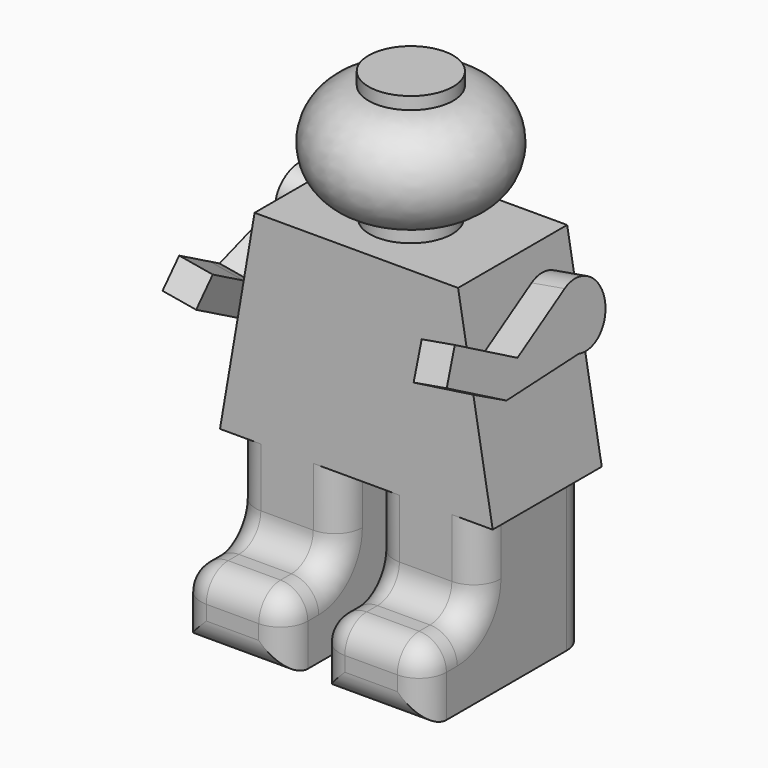
from build123d import *

# Parameters (mm, degrees)
F0_W      = 19.9313152116
F0_H      = 28.9478618652
F1_DEPTH  = 12.7
F2_W      = 19.9313152116
F2_H      = 12.9078961909
F3_DEPTH  = 12.7
F4_F1_R   = 5.08
F4_F2_R   = 5.08
F8_DEPTH  = 6.2511
F10_DEPTH = 6.35


with BuildPart() as f1:
    # F0 (on Front) → F1 (new body, symmetric)
    with BuildSketch(Plane.XZ):
        Polygon((22.873558104, 0), (25.4, 0), (18.9548347086, 37.5508967185), (0, 37.5508967185), (0, 0), (2.9422428925, 0), align=None)
        with Locations((12.9079004982, -14.4739309326)):
            Rectangle(F0_W, F0_H)
        Polygon((0, 0), (0, 37.5508967185), (-18.9548347086, 37.5508967185), (-25.4, 0), (-22.873558104, 0), (-2.9422428925, 0), align=None)
        with Locations((-12.9079004982, -14.4739309326)):
            Rectangle(F0_W, F0_H)
    extrude(amount=F1_DEPTH, both=True)

    # F2 (on face) → F3 (join)
    with BuildSketch(Plane.XZ.offset(12.7)):
        with Locations((12.9079004982, -22.4939137697)):
            Rectangle(F2_W, F2_H)
        with Locations((-12.9079004982, -22.4939137697)):
            Rectangle(F2_W, F2_H)
    extrude(amount=F3_DEPTH)

    # F4: fillet of radius 5.08 on 18 edges, made by hand

    # F4_f1
    f4_f1_edges = [f1.edges().sort_by_distance(p)[0] for p in [
        (12.9079004982, -12.7, -16.0399656743),
        (-12.9079004982, -12.7, -16.0399656743),
    ]]
    fillet(f4_f1_edges, radius=F4_F1_R)

    # F4_f2
    f4_f2_edges = [f1.edges().sort_by_distance(p)[0] for p in [
        (-2.9422428925, -25.4, -22.4939137697),
        (-12.9079004982, -25.4, -16.0399656743),
        (-22.873558104, -25.4, -22.4939137697),
        (-12.9079004982, -25.4, -28.9478618652),
        (22.873558104, -25.4, -22.4939137697),
        (12.9079004982, -25.4, -16.0399656743),
        (2.9422428925, -25.4, -22.4939137697),
        (12.9079004982, -25.4, -28.9478618652),
        (-2.9422428925, -21.59, -16.0399656743),
        (-22.873558104, -21.59, -16.0399656743),
        (22.873558104, 12.7, -14.4739309326),
        (2.9422428925, 12.7, -14.4739309326),
        (-22.873558104, 12.7, -14.4739309326),
        (-2.9422428925, 12.7, -14.4739309326),
        (22.873558104, -12.7, -5.4799828371),
        (2.9422428925, -12.7, -5.4799828371),
        (2.9422428925, -14.1878975516, -14.5520681227),
        (22.873558104, -14.1878975516, -14.5520681227),
        (-22.873558104, -14.1878975516, -14.5520681227),
        (-2.9422428925, -14.1878975516, -14.5520681227),
    ]]
    fillet(f4_f2_edges, radius=F4_F2_R)

    # F5 (on Front) → F6 (revolve)
    with BuildSketch(Plane.XZ):
        with BuildLine():
            Line((7.6877931133, 33.1239514053), (7.6877931133, 40.7419648703))
            ThreePointArc((7.6877931133, 40.7419648703), (16.6857685514, 50.0178025185), (7.8776162118, 59.4740797153))
            Line((7.8776162118, 59.4740797153), (7.8776162118, 61.787083745))
            Line((7.8776162118, 61.787083745), (0, 61.787083745))
            Line((0, 61.787083745), (0, 33.1239514053))
            Line((0, 33.1239514053), (7.6877931133, 33.1239514053))
        make_face()
    revolve(axis=Axis((0, 0, 47.4555175751), (0, 0, 1)))

    # F7 (on face) → F8 (join)
    with BuildSketch(Plane(origin=(24.6731381341, 0, 4.234851027), x_dir=(0, 1, 0), z_dir=(0.9855878404, 0, 0.1691644433))):
        with BuildLine():
            Line((-12.7, 16.9602958167), (4.2709973641, 17.6954660565))
            ThreePointArc((4.2709973641, 17.6954660565), (11.5417566939, 23.7592524776), (3.2686796257, 28.3624733953))
            Line((3.2686796257, 28.3624733953), (-9.0165464208, 22.251194343))
            Line((-9.0165464208, 22.251194343), (-22.1028998209, 29.3900118281))
            Line((-22.1028998209, 29.3900118281), (-25.1719959147, 23.7639713547))
            Line((-25.1719959147, 23.7639713547), (-12.7, 16.9602958167))
        make_face()
    extrude(amount=F8_DEPTH)

    # F9 (on face) → F10 (join)
    with BuildSketch(Plane(origin=(-24.6731381341, 0, 4.234851027), x_dir=(0, -1, 0), z_dir=(-0.9855878404, 0, 0.1691644433))):
        with BuildLine():
            Line((10.2126034461, 20.4402103872), (-1.7259411979, 25.6970115006))
            ThreePointArc((-1.7259411979, 25.6970115006), (-8.7725675478, 30.2032799266), (-6.2509044074, 22.2281552851))
            Line((-6.2509044074, 22.2281552851), (10.7428459451, 14.1681702808))
            Line((10.7428459451, 14.1681702808), (12.7, 15.2765091522))
            Line((12.7, 15.2765091522), (12.7, 21.8488262713))
            Line((12.7, 21.8488262713), (10.2126034461, 20.4402103872))
        make_face()
        Polygon((20.8962647478, 26.4903815939), (12.7, 21.8488262713), (12.7, 15.2765091522), (23.7144064158, 21.5139817446), align=None)
    extrude(amount=F10_DEPTH)


solid = f1.part
